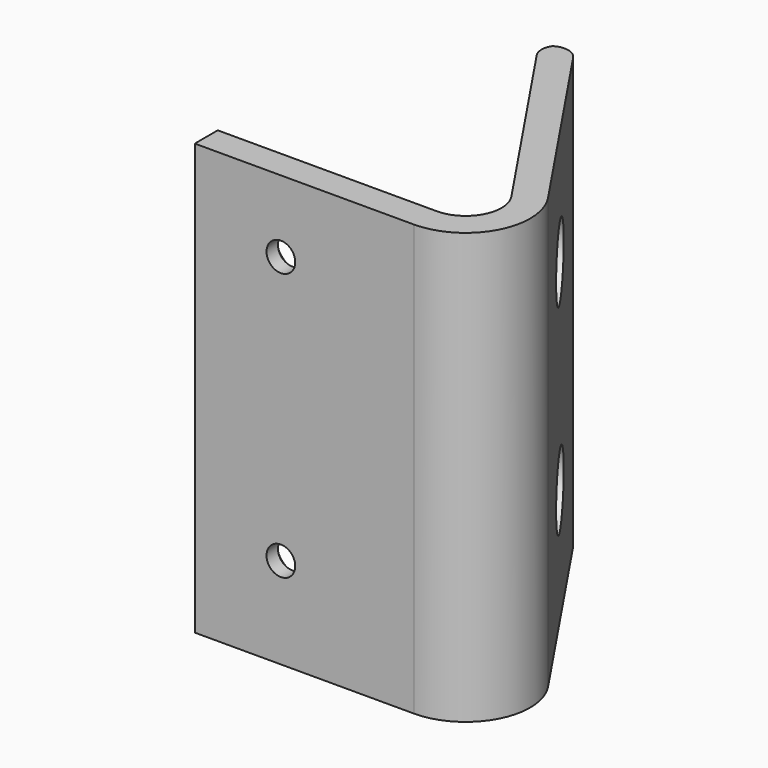
from build123d import *

# Parameters (mm, degrees)
F1_DEPTH    = 60
F2_R        = 5
F3_DEPTH    = 25
F4_R        = 2
F5_DEPTH    = 25
F6_SIZE     = 2
F7_SIZE     = 2
F8_R        = 2.5
F9_T1_DEPTH = 71.4564392374


# Not quite as in the source:
# - a fillet or chamfer that OpenCascade refuses, or shapes differently, is made with other operations: its cross-section is extruded or revolved along the edge and cut away or added


with BuildPart() as f1:
    # F0 (on Top) → F1 (new body)
    with BuildSketch(Plane.XY):
        with BuildLine():
            Line((0, 4), (0, 0))
            Line((0, 0), (30.5437369547, 0))
            ThreePointArc((30.5437369547, 0), (38.4878384458, 4.7701948627), (38.0108483544, 14.0241663334))
            Line((38.0108483544, 14.0241663334), (18.0912535296, 43.6294428556))
            Line((18.0912535296, 43.6294428556), (14.7725373519, 41.3964800408))
            Line((14.7725373519, 41.3964800408), (33.0393692072, 14.2476041216))
            Line((33.0393692072, 14.2476041216), (34.6921321767, 11.7912035185))
            ThreePointArc((34.6921321767, 11.7912035185), (34.957126672, 6.650108257), (30.5437369547, 4))
            Line((30.5437369547, 4), (0, 4))
        make_face()
    extrude(amount=F1_DEPTH)

    # F2 (on face) → F3 (cut)
    with BuildSketch(Plane(origin=(32.6608671723, 21.9755164324, 0), x_dir=(-0.5582407037, 0.8296790444, 0), z_dir=(0.8296790444, 0.5582407037, 0))):
        with Locations((6.0991603551, 44)):
            Circle(F2_R)
        with Locations((6.0991603551, 16)):
            Circle(F2_R)
    extrude(amount=-F3_DEPTH, mode=Mode.SUBTRACT)

    # F4 (on face) → F5 (cut)
    with BuildSketch(Plane.XZ):
        with Locations((12, 12.7154784277)):
            Circle(F4_R)
        with Locations((12, 50)):
            Circle(F4_R)
    extrude(amount=-F5_DEPTH, mode=Mode.SUBTRACT)

    # F6
    f6_edges = [f1.edges().sort_by_distance(p)[0] for p in [
        (10, 4, 12.715478),
    ]]
    chamfer(f6_edges, length=F6_SIZE)

    # F7
    f7_edges = [f1.edges().sort_by_distance(p)[0] for p in [
        (10, 4, 50),
    ]]
    chamfer(f7_edges, length=F7_SIZE)

    # F8
    f8_edges = [f1.edges().sort_by_distance(p)[0] for p in [
        (18.091254, 43.629443, 30),
    ]]
    fillet(f8_edges, radius=F8_R)

    # F9: fillet of radius 2.5 on 1 edges, made by hand

    # F9_s2 → F9_t1 (cut)
    with BuildSketch(Plane.XY.offset(-5.7282196187)):
        with BuildLine():
            ThreePointArc((16.0170559185, 42.2338410964), (15.6260243102, 40.8594889036), (16.0516274923, 39.495446529))
            Line((16.0516274923, 39.495446529), (14.7725373519, 41.3964800408))
            Line((14.7725373519, 41.3964800408), (16.0170559185, 42.2338410964))
        make_face()
    extrude(amount=F9_T1_DEPTH, mode=Mode.SUBTRACT)


solid = f1.part
